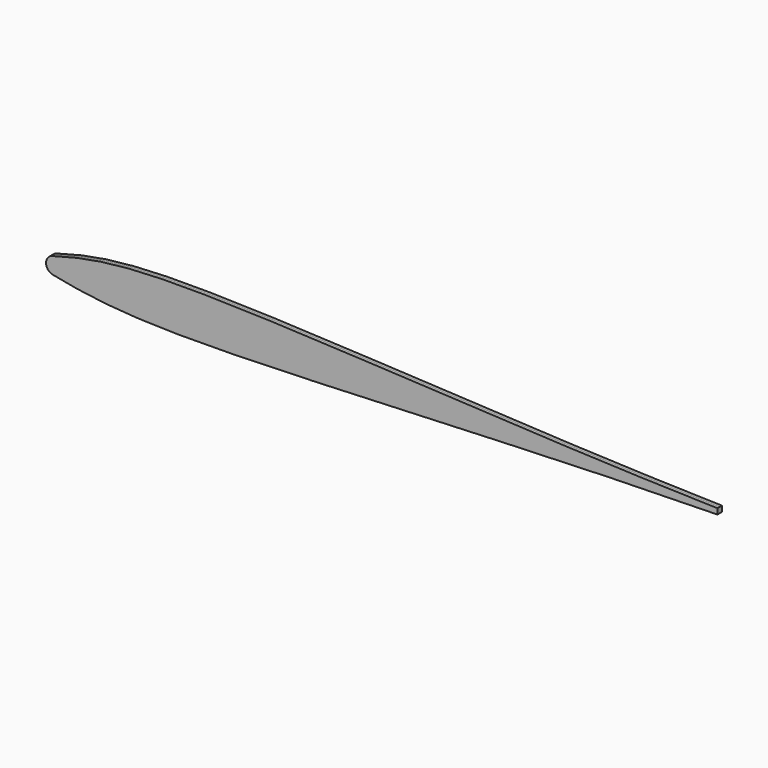
from build123d import *

# Parameters (mm, degrees)
F0_R     = 2.2
F1_DEPTH = 0.5


# Not quite as in the source:
# - a feature names something its author has since deleted; it is built from what else it names


with BuildPart() as f1:
    # F0 (on Front) → F1 (new body, symmetric)
    with BuildSketch(Plane.XZ):
        with BuildLine():
            add(Edge.make_bspline(
                [(-58.9228828544, 1.4755374035), (-53.1031861901, 3.1954683363), (-35.6327797164, 6.0866905267), (21.0318658501, 1.3725945028), (60.0087855716, 0.4661711108)],
                knots=[0, 0, 0, 0, 0.3159620499, 1, 1, 1, 1], degree=3))
            ThreePointArc((-58.9228828544, 1.4755374035), (-60.0086458958, 0.0133592085), (-58.8833838701, -1.4186435253))
            add(Edge.make_bspline(
                [(-58.8833838701, -1.4186435253), (-53.4330829978, -2.5445383508), (-35.3326671897, -5.1505314866), (21.6348022223, -1.0668247705), (60.0087855716, -0.5338288892)],
                knots=[0, 0, 0, 0, 0.3153766332, 1, 1, 1, 1], degree=3))
            Line((60.0087855716, -0.5338288892), (60.0087855716, -0.0338288892))
            Line((60.0087855716, -0.0338288892), (60.0087855716, 0.4661711108))
        make_face()
        with BuildLine():
            add(Edge.make_bspline(
                [(-38.2616780698, 3.6168415099), (-37.3862738566, 3.620107016), (-36.5051030136, 3.6204740501), (-35.618541931, 3.6180910206)],
                knots=[0, 0, 0, 0, 2.8040999397, 2.8040999397, 2.8040999397, 2.8040999397], degree=3))
            add(Edge.make_bspline(
                [(-35.618541931, 3.6180910206), (-28.2361493541, 3.598247538), (-20.4800034879, 3.3877176683), (-12.5674262287, 3.0721900892)],
                knots=[2.8040999397, 2.8040999397, 2.8040999397, 2.8040999397, 26.1538352096, 26.1538352096, 26.1538352096, 26.1538352096], degree=3))
            add(Edge.make_bspline(
                [(-12.5674262287, 3.0721900892), (-12.2191674657, 3.0583026741), (-11.8706056681, 3.0442118605), (-11.5217593652, 3.0299249541)],
                knots=[26.1538352096, 26.1538352096, 26.1538352096, 26.1538352096, 27.1815344858, 27.1815344858, 27.1815344858, 27.1815344858], degree=3))
            add(Edge.make_bspline(
                [(-11.5217593652, 3.0299249541), (-4.8786493859, 2.7578581748), (1.8676333595, 2.4146805186), (8.5891307931, 2.0508450631)],
                knots=[27.1815344858, 27.1815344858, 27.1815344858, 27.1815344858, 46.7520996913, 46.7520996913, 46.7520996913, 46.7520996913], degree=3))
            add(Edge.make_bspline(
                [(8.5891307931, 2.0508450631), (8.9659043148, 2.0304502675), (9.3425999571, 2.0099905618), (9.7191951821, 1.9894748324)],
                knots=[46.7520996913, 46.7520996913, 46.7520996913, 46.7520996913, 47.8491276748, 47.8491276748, 47.8491276748, 47.8491276748], degree=3))
            add(Edge.make_bspline(
                [(9.7191951821, 1.9894748324), (22.9972566346, 1.2661275955), (36.1504854864, 0.4731351449), (48.1910333037, 0)],
                knots=[47.8491276748, 47.8491276748, 47.8491276748, 47.8491276748, 86.5283355113, 86.5283355113, 86.5283355113, 86.5283355113], degree=3))
            add(Edge.make_bspline(
                [(9.7191951821, -1.4306571949), (23.0872151546, -0.8738704636), (36.291554297, -0.3020974887), (48.1910333037, 0)],
                knots=[47.589168745, 47.589168745, 47.589168745, 47.589168745, 86.3670691529, 86.3670691529, 86.3670691529, 86.3670691529], degree=3))
            add(Edge.make_bspline(
                [(8.5891307931, -1.4776679077), (8.9659317989, -1.4620138036), (9.3426284313, -1.4463414451), (9.7191951821, -1.4306571949)],
                knots=[46.4968253771, 46.4968253771, 46.4968253771, 46.4968253771, 47.589168745, 47.589168745, 47.589168745, 47.589168745], degree=3))
            add(Edge.make_bspline(
                [(-8.0119146338, -2.1358759001), (-2.5096790564, -1.9338850607), (3.0509994649, -1.7077481956), (8.5891307931, -1.4776679077)],
                knots=[30.4418230465, 30.4418230465, 30.4418230465, 30.4418230465, 46.4968253771, 46.4968253771, 46.4968253771, 46.4968253771], degree=3))
            add(Edge.make_bspline(
                [(-9.1685029524, -2.1780045759), (-8.7832794964, -2.1640850551), (-8.3977407486, -2.1500398412), (-8.0119146338, -2.1358759001)],
                knots=[29.3160189827, 29.3160189827, 29.3160189827, 29.3160189827, 30.4418230465, 30.4418230465, 30.4418230465, 30.4418230465], degree=3))
            add(Edge.make_bspline(
                [(-16.1278416778, -2.4155654967), (-13.8237679533, -2.3420223971), (-11.5019196333, -2.262319385), (-9.1685029524, -2.1780045759)],
                knots=[22.4966783089, 22.4966783089, 22.4966783089, 22.4966783089, 29.3160189827, 29.3160189827, 29.3160189827, 29.3160189827], degree=3))
            add(Edge.make_bspline(
                [(-17.6034438118, -2.4618844422), (-17.1124296707, -2.4467365601), (-16.620542064, -2.4312918657), (-16.1278416778, -2.4155654967)],
                knots=[21.0384386058, 21.0384386058, 21.0384386058, 21.0384386058, 22.4966783089, 22.4966783089, 22.4966783089, 22.4966783089], degree=3))
            add(Edge.make_bspline(
                [(-35.618541931, -2.8627375282), (-29.832875954, -2.7963595375), (-23.7874330759, -2.6526617177), (-17.6034438118, -2.4618844422)],
                knots=[2.6729010132, 2.6729010132, 2.6729010132, 2.6729010132, 21.0384386058, 21.0384386058, 21.0384386058, 21.0384386058], degree=3))
            add(Edge.make_bspline(
                [(-38.1277799606, -2.8867127839), (-37.2971189192, -2.8804209375), (-36.4605816684, -2.8723981111), (-35.618541931, -2.8627375282)],
                knots=[0, 0, 0, 0, 2.6729010132, 2.6729010132, 2.6729010132, 2.6729010132], degree=3))
            add(Edge.make_bspline(
                [(-41.2343927197, -2.813945704), (-40.1954922608, -2.8458899458), (-39.1588154774, -2.8693293605), (-38.1277799606, -2.8867127839)],
                knots=[17.7850046696, 17.7850046696, 17.7850046696, 17.7850046696, 20.8486920648, 20.8486920648, 20.8486920648, 20.8486920648], degree=3))
            add(Edge.make_bspline(
                [(-58.8833838701, -0.9187526302), (-53.3711660516, -2.1564612924), (-47.2653113899, -2.6285062592), (-41.2343927197, -2.813945704)],
                knots=[0, 0, 0, 0, 17.7850046696, 17.7850046696, 17.7850046696, 17.7850046696], degree=3))
            ThreePointArc((-58.8833838701, -0.9187526302), (-59.3690674128, 0.0570033976), (-58.9228828544, 1.0514417663))
            add(Edge.make_bspline(
                [(-58.9228828544, 1.0514417663), (-53.1244599749, 2.7082601042), (-46.8471278917, 3.3047021461), (-41.2402659449, 3.5280295404)],
                knots=[0, 0, 0, 0, 17.6226858026, 17.6226858026, 17.6226858026, 17.6226858026], degree=3))
            add(Edge.make_bspline(
                [(-41.2402659449, 3.5280295404), (-40.2230472035, 3.5685464665), (-39.2278967387, 3.5967824619), (-38.2616780698, 3.6168415099)],
                knots=[17.6226858026, 17.6226858026, 17.6226858026, 17.6226858026, 20.8198621272, 20.8198621272, 20.8198621272, 20.8198621272], degree=3))
        make_face(mode=Mode.SUBTRACT)
        with BuildLine():
            add(Edge.make_bspline(
                [(-35.618541931, 3.6180910206), (-28.2361493541, 3.598247538), (-20.4800034879, 3.3877176683), (-12.5674262287, 3.0721900892)],
                knots=[2.8040999397, 2.8040999397, 2.8040999397, 2.8040999397, 26.1538352096, 26.1538352096, 26.1538352096, 26.1538352096], degree=3))
            Line((-35.618541931, 3.6180910206), (-35.618541931, -2.8627375282))
            add(Edge.make_bspline(
                [(-35.618541931, -2.8627375282), (-29.832875954, -2.7963595375), (-23.7874330759, -2.6526617177), (-17.6034438118, -2.4618844422)],
                knots=[2.6729010132, 2.6729010132, 2.6729010132, 2.6729010132, 21.0384386058, 21.0384386058, 21.0384386058, 21.0384386058], degree=3))
            Line((-17.6034438118, -2.4618844422), (-12.5674262287, 3.0721900892))
        make_face()
        with BuildLine():
            Line((-41.2343927197, -2.813945704), (-41.2402659449, 3.5280295404))
            add(Edge.make_bspline(
                [(-58.9228828544, 1.0514417663), (-53.1244599749, 2.7082601042), (-46.8471278917, 3.3047021461), (-41.2402659449, 3.5280295404)],
                knots=[0, 0, 0, 0, 17.6226858026, 17.6226858026, 17.6226858026, 17.6226858026], degree=3))
            ThreePointArc((-58.9228828544, 1.0514417663), (-59.3690674128, 0.0570033976), (-58.8833838701, -0.9187526302))
            add(Edge.make_bspline(
                [(-58.8833838701, -0.9187526302), (-53.3711660516, -2.1564612924), (-47.2653113899, -2.6285062592), (-41.2343927197, -2.813945704)],
                knots=[0, 0, 0, 0, 17.7850046696, 17.7850046696, 17.7850046696, 17.7850046696], degree=3))
        make_face()
        with BuildLine():
            add(Edge.make_bspline(
                [(-11.5217593652, 3.0299249541), (-4.8786493859, 2.7578581748), (1.8676333595, 2.4146805186), (8.5891307931, 2.0508450631)],
                knots=[27.1815344858, 27.1815344858, 27.1815344858, 27.1815344858, 46.7520996913, 46.7520996913, 46.7520996913, 46.7520996913], degree=3))
            Line((-11.5217593652, 3.0299249541), (-8.0119146338, -2.1358759001))
            add(Edge.make_bspline(
                [(-8.0119146338, -2.1358759001), (-2.5096790564, -1.9338850607), (3.0509994649, -1.7077481956), (8.5891307931, -1.4776679077)],
                knots=[30.4418230465, 30.4418230465, 30.4418230465, 30.4418230465, 46.4968253771, 46.4968253771, 46.4968253771, 46.4968253771], degree=3))
            Line((8.5891307931, -1.4776679077), (8.5891307931, 2.0508450631))
        make_face()
        with BuildLine():
            add(Edge.make_bspline(
                [(9.7191951821, 1.9894748324), (22.9972566346, 1.2661275955), (36.1504854864, 0.4731351449), (48.1910333037, 0)],
                knots=[47.8491276748, 47.8491276748, 47.8491276748, 47.8491276748, 86.5283355113, 86.5283355113, 86.5283355113, 86.5283355113], degree=3))
            Line((9.7191951821, 1.9894748324), (9.7191951821, -1.4306571949))
            add(Edge.make_bspline(
                [(9.7191951821, -1.4306571949), (23.0872151546, -0.8738704636), (36.291554297, -0.3020974887), (48.1910333037, 0)],
                knots=[47.589168745, 47.589168745, 47.589168745, 47.589168745, 86.3670691529, 86.3670691529, 86.3670691529, 86.3670691529], degree=3))
        make_face()
        with BuildLine():
            Line((-35.618541931, -2.8627375282), (-35.618541931, 3.6180910206))
            add(Edge.make_bspline(
                [(-38.2616780698, 3.6168415099), (-37.3862738566, 3.620107016), (-36.5051030136, 3.6204740501), (-35.618541931, 3.6180910206)],
                knots=[0, 0, 0, 0, 2.8040999397, 2.8040999397, 2.8040999397, 2.8040999397], degree=3))
            add(Edge.make_bspline(
                [(-41.2402659449, 3.5280295404), (-40.2230472035, 3.5685464665), (-39.2278967387, 3.5967824619), (-38.2616780698, 3.6168415099)],
                knots=[17.6226858026, 17.6226858026, 17.6226858026, 17.6226858026, 20.8198621272, 20.8198621272, 20.8198621272, 20.8198621272], degree=3))
            Line((-41.2402659449, 3.5280295404), (-41.2343927197, -2.813945704))
            add(Edge.make_bspline(
                [(-41.2343927197, -2.813945704), (-40.1954922608, -2.8458899458), (-39.1588154774, -2.8693293605), (-38.1277799606, -2.8867127839)],
                knots=[17.7850046696, 17.7850046696, 17.7850046696, 17.7850046696, 20.8486920648, 20.8486920648, 20.8486920648, 20.8486920648], degree=3))
            add(Edge.make_bspline(
                [(-38.1277799606, -2.8867127839), (-37.2971189192, -2.8804209375), (-36.4605816684, -2.8723981111), (-35.618541931, -2.8627375282)],
                knots=[0, 0, 0, 0, 2.6729010132, 2.6729010132, 2.6729010132, 2.6729010132], degree=3))
        make_face()
        with Locations((-38.368541931, 0.4547677818)):
            Circle(F0_R, mode=Mode.SUBTRACT)
        with Locations((-38.368541931, 0.4547677818)):
            Circle(F0_R)
        with BuildLine():
            Line((-12.0510029943, 2.0644683304), (-16.1278416778, -2.4155654967))
            add(Edge.make_bspline(
                [(-16.1278416778, -2.4155654967), (-13.8237679533, -2.3420223971), (-11.5019196333, -2.262319385), (-9.1685029524, -2.1780045759)],
                knots=[22.4966783089, 22.4966783089, 22.4966783089, 22.4966783089, 29.3160189827, 29.3160189827, 29.3160189827, 29.3160189827], degree=3))
            Line((-9.1685029524, -2.1780045759), (-12.0510029943, 2.0644683304))
        make_face()
        with BuildLine():
            add(Edge.make_bspline(
                [(-12.5674262287, 3.0721900892), (-12.2191674657, 3.0583026741), (-11.8706056681, 3.0442118605), (-11.5217593652, 3.0299249541)],
                knots=[26.1538352096, 26.1538352096, 26.1538352096, 26.1538352096, 27.1815344858, 27.1815344858, 27.1815344858, 27.1815344858], degree=3))
            Line((-12.5674262287, 3.0721900892), (-17.6034438118, -2.4618844422))
            add(Edge.make_bspline(
                [(-17.6034438118, -2.4618844422), (-17.1124296707, -2.4467365601), (-16.620542064, -2.4312918657), (-16.1278416778, -2.4155654967)],
                knots=[21.0384386058, 21.0384386058, 21.0384386058, 21.0384386058, 22.4966783089, 22.4966783089, 22.4966783089, 22.4966783089], degree=3))
            Line((-16.1278416778, -2.4155654967), (-12.0510029943, 2.0644683304))
            Line((-12.0510029943, 2.0644683304), (-9.1685029524, -2.1780045759))
            add(Edge.make_bspline(
                [(-9.1685029524, -2.1780045759), (-8.7832794964, -2.1640850551), (-8.3977407486, -2.1500398412), (-8.0119146338, -2.1358759001)],
                knots=[29.3160189827, 29.3160189827, 29.3160189827, 29.3160189827, 30.4418230465, 30.4418230465, 30.4418230465, 30.4418230465], degree=3))
            Line((-8.0119146338, -2.1358759001), (-11.5217593652, 3.0299249541))
        make_face()
        with BuildLine():
            add(Edge.make_bspline(
                [(8.5891307931, 2.0508450631), (8.9659043148, 2.0304502675), (9.3425999571, 2.0099905618), (9.7191951821, 1.9894748324)],
                knots=[46.7520996913, 46.7520996913, 46.7520996913, 46.7520996913, 47.8491276748, 47.8491276748, 47.8491276748, 47.8491276748], degree=3))
            Line((8.5891307931, 2.0508450631), (8.5891307931, -1.4776679077))
            add(Edge.make_bspline(
                [(8.5891307931, -1.4776679077), (8.9659317989, -1.4620138036), (9.3426284313, -1.4463414451), (9.7191951821, -1.4306571949)],
                knots=[46.4968253771, 46.4968253771, 46.4968253771, 46.4968253771, 47.589168745, 47.589168745, 47.589168745, 47.589168745], degree=3))
            Line((9.7191951821, -1.4306571949), (9.7191951821, 1.9894748324))
        make_face()
    extrude(amount=F1_DEPTH, both=True)


solid = f1.part
